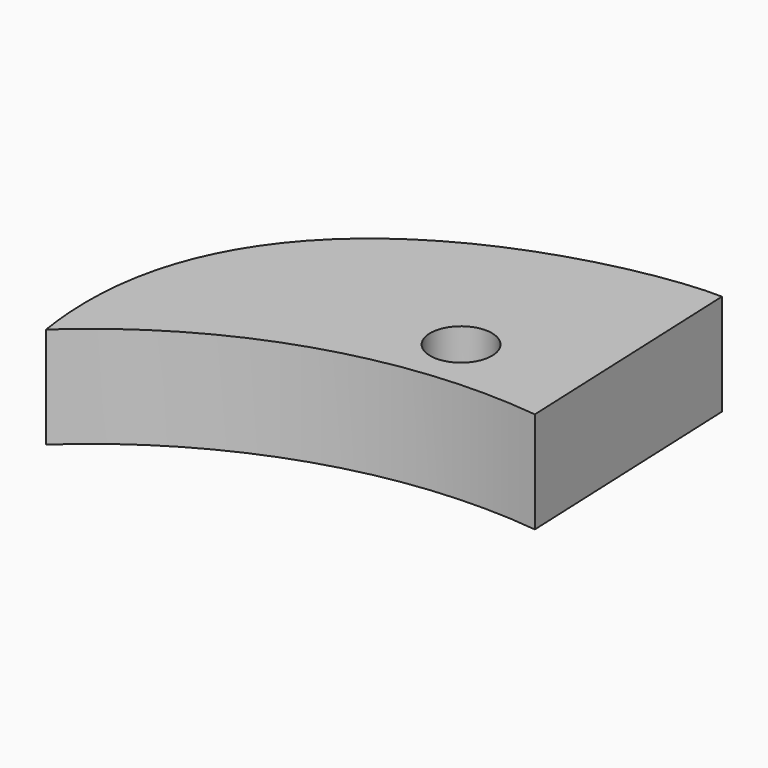
from build123d import *

# Parameters (mm, degrees)
F0_R     = 3.0930971136
F1_DEPTH = 10.16


# Not quite as in the source:
# - a feature names something its author has since deleted; it is built from what else it names


with BuildPart() as f1:
    # F0 (on Top) → F1 (new body)
    with BuildSketch(Plane.XY):
        with BuildLine():
            Line((11.9163581484, 0), (10.8801536262, 24.745227769))
            add(Edge.make_bspline(
                [(10.8801536262, 24.745227769), (2.5768475607, 25.0708498061), (-31.8439677358, 18.5879450291), (-26.9596707076, -12.6715619117)],
                knots=[0, 0, 0, 0, 53.2153028331, 53.2153028331, 53.2153028331, 53.2153028331], degree=3))
            ThreePointArc((-26.9596707076, -12.6715619117), (-8.9067406272, -2.0863774931), (11.9163581484, 0))
        make_face()
        with Locations((0, 5.6472551078)):
            Circle(F0_R, mode=Mode.SUBTRACT)
    extrude(amount=F1_DEPTH)


solid = f1.part
